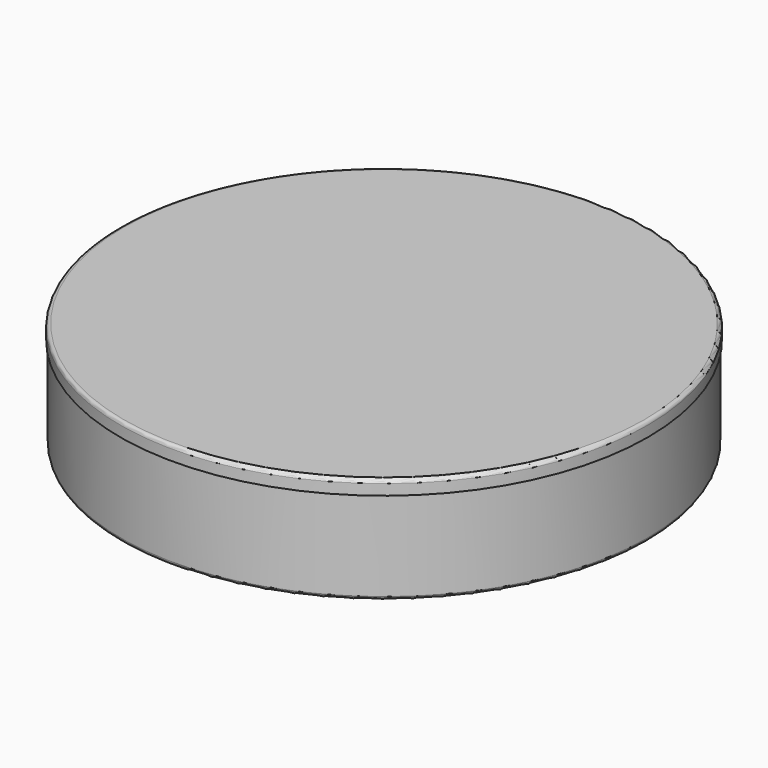
from build123d import *

# Parameters (mm, degrees)
F0_R     = 36.75
F0_R_2   = 35.75
F1_DEPTH = 15
F2_R     = 36.9218427358
F3_DEPTH = 2
F4_R     = 0.49999


# Not quite as in the source:
# - a fillet or chamfer is up to 0.001 mm smaller than in the source, because OpenCascade refuses the exact size


with BuildPart() as f1:
    # F0 (on Top) → F1 (new body)
    with BuildSketch(Plane.XY):
        Circle(F0_R)
        Circle(F0_R_2, mode=Mode.SUBTRACT)
    extrude(amount=F1_DEPTH)

    # F2 (on face) → F3 (join)
    with BuildSketch(Plane.XY.offset(15)):
        Circle(F2_R)
    extrude(amount=-F3_DEPTH)

    # F4 (radius 0.5 in the source; OpenCascade refuses exactly that, so slightly less here)
    f4_edges = [f1.edges().sort_by_distance(p)[0] for p in [
        (-36.75, 0, 0),
        (-35.75, 0, 0),
        (-36.921843, 0, 15),
    ]]
    fillet(f4_edges, radius=F4_R)


solid = f1.part
